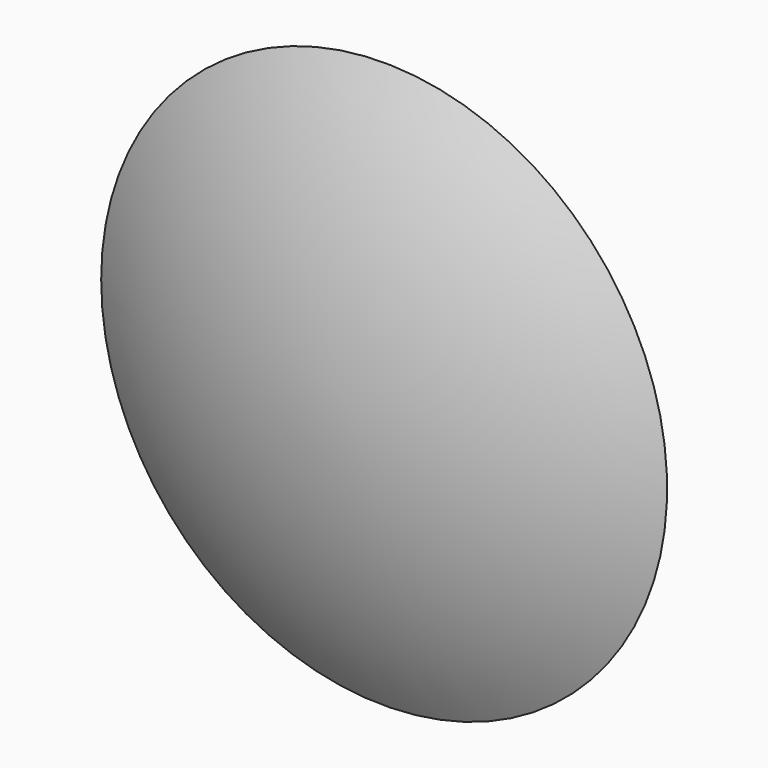
from build123d import *


# Not quite as in the source:
# - the program builds the solid bodies; features that only make, move or delete a surface that nothing else refers to are left out


with BuildPart() as f2:
    # F0 (on Top) → F2 (revolve)
    with BuildSketch(Plane.XY):
        with BuildLine():
            Line((0, -16.6293936748), (0, -12.7))
            Line((0, -12.7), (-14.6646968374, -12.7))
            ThreePointArc((-14.6646968374, -12.7), (-7.5910056644, -15.6300188199), (0, -16.6293936748))
        make_face()
    revolve(axis=Axis((0, -14.6646968374, 0), (0, -1, 0)))


solid = f2.part
